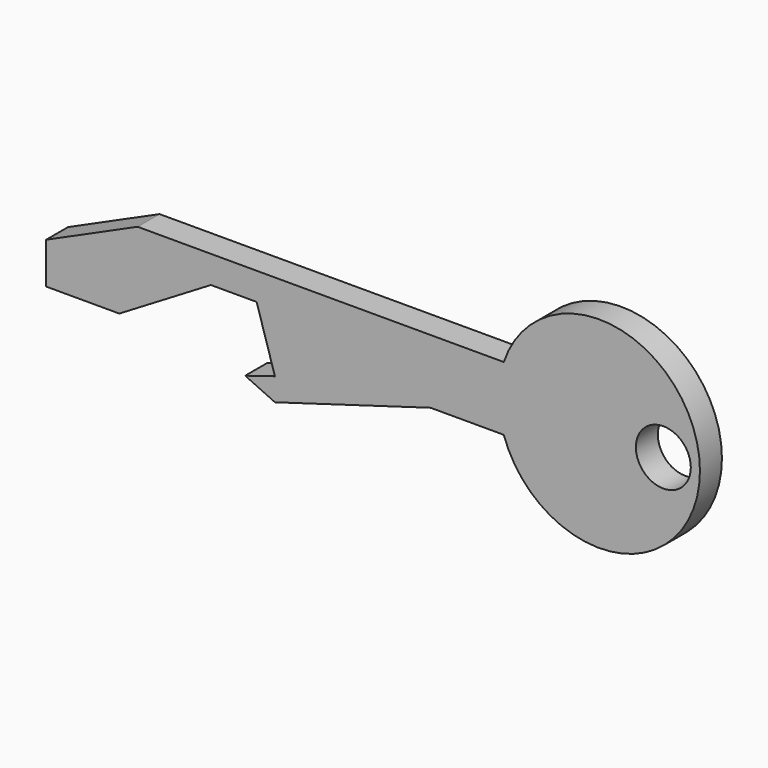
from build123d import *

# Parameters (mm, degrees)
F0_R     = 3
F1_DEPTH = 3


# Not quite as in the source:
# - a feature names something its author has since deleted; it is built from what else it names


with BuildPart() as f1:
    # F0 (on Front) → F1 (new body)
    with BuildSketch(Plane.XZ):
        Polygon((-2, -2), (1.3333333333, 0), (0, 0), (0, 7), (-10, 2.5), (-10, -2), align=None)
        Polygon((14.2307692308, 0), (32, 0), (40, 0), (40, 7), (0, 7), (0, 0), (1.3333333333, 0), (8, 4), (13, 4), align=None)
        Polygon((15, -5), (32, 0), (14.2307692308, 0), (15, -2.5), (11.75, -3.5), align=None)
        with BuildLine():
            Line((40, 7), (40, 0))
            ThreePointArc((40, 0), (61.4283268073, 3.5), (40, 7))
        make_face()
        with Locations((57.4283268073, 3.5)):
            Circle(F0_R, mode=Mode.SUBTRACT)
    extrude(amount=F1_DEPTH)


solid = f1.part
